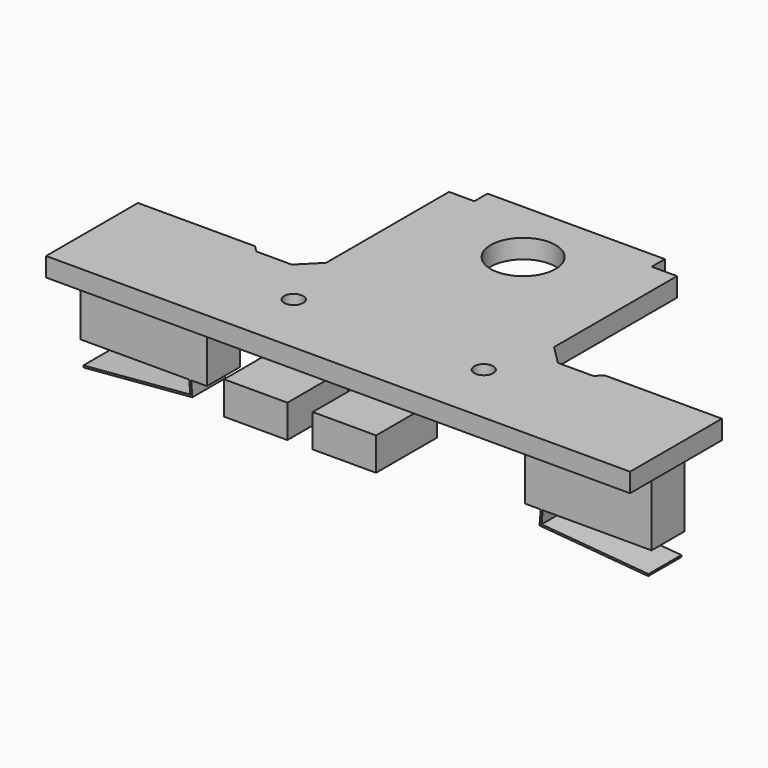
from build123d import *

# Parameters (mm, degrees)
F0_R     = 1.5
F0_R_2   = 5.125
F1_DEPTH = 3
F2_W     = 20
F2_H     = 6.5
F3_DEPTH = 10.5
F5_DEPTH = 6.5
F6_W     = 16
F6_H     = 4.5
F7_DEPTH = 5.7
F8_W     = 10
F8_H     = 12
F9_DEPTH = 5.2


# Not quite as in the source:
# - a pattern or mirror of a feature is missing from the dataset's text; its kind, count and spacing are read off the source's solid


with BuildPart() as f1:
    # F0 (on Top) → F1 (new body)
    with BuildSketch(Plane.XY):
        Polygon((-46.1, 18.13), (-46.1, 0), (46.1, 0), (46.1, 18.13), (27.6, 18.13), (26.6, 17.13), (21, 17.13), (18, 20.13), (18, 44.4), (14, 44.4), (14, 47), (-14, 47), (-14, 44.4), (-18, 44.4), (-18, 20.13), (-21, 17.13), (-26.6, 17.13), (-27.6, 18.13), align=None)
        with Locations((-15, 10)):
            Circle(F0_R, mode=Mode.SUBTRACT)
        with Locations((15, 10)):
            Circle(F0_R, mode=Mode.SUBTRACT)
        with Locations((0, 36.525)):
            Circle(F0_R_2, mode=Mode.SUBTRACT)
    extrude(amount=F1_DEPTH)

    # F2 (on face) → F3 (join)
    with BuildSketch(Plane(origin=(0, 0, 0), x_dir=(1, 0, 0), z_dir=(0, 0, -1))):
        with Locations((-35.1, -8.75)):
            Rectangle(F2_W, F2_H)
    f3 = extrude(amount=F3_DEPTH)

    # F3_copies: F3 across plane
    add(f3.mirror(Plane(origin=(0, 0, 0), x_dir=(0, 0, 1), z_dir=(1, 0, 0))))

    # F4 (on face) → F5 (join, through all)
    with BuildSketch(Plane(origin=(0, 12, 0), x_dir=(-1, 0, 0), z_dir=(0, 1, 0))):
        Polygon((44.5747535126, -14.25), (44.6, -13.9510641961), (27.7299368373, -12.5263106834), (27.9010679845, -10.5), (27.6, -10.5), (27.4057545459, -12.8), align=None)
    f5 = extrude(amount=-F5_DEPTH)

    # F5_copies: F5 across plane
    add(f5.mirror(Plane(origin=(0, 0, 0), x_dir=(0, 0, 1), z_dir=(1, 0, 0))))

    # F6 (on face) → F7 (join)
    with BuildSketch(Plane(origin=(0, 0, 0), x_dir=(1, 0, 0), z_dir=(0, 0, -1))):
        with Locations((0, -10.25)):
            Rectangle(F6_W, F6_H)
    extrude(amount=F7_DEPTH)

    # F8 (on face) → F9 (join)
    with BuildSketch(Plane(origin=(0, 0, 0), x_dir=(1, 0, 0), z_dir=(0, 0, -1))):
        with Locations((-7, 1.5)):
            Rectangle(F8_W, F8_H)
        with Locations((7, 1.5)):
            Rectangle(F8_W, F8_H)
    extrude(amount=F9_DEPTH)


solid = f1.part
